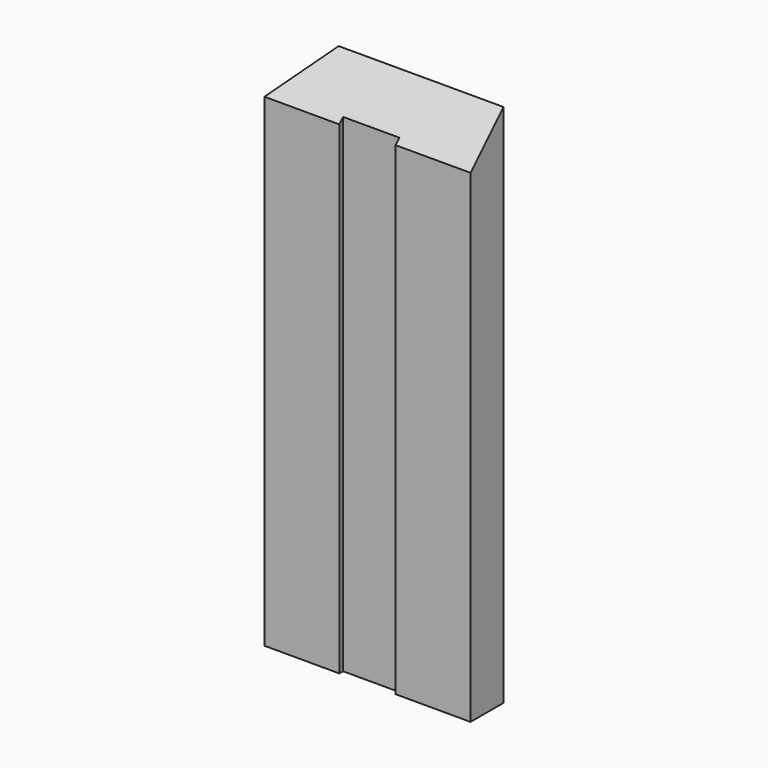
from build123d import *

# Parameters (mm, degrees)
F0_W     = 139.7
F0_H     = 27.94
F1_DEPTH = 355.6
F2_SIZE  = 27.93999
F3_W     = 38.1
F3_H     = 355.6
F4_DEPTH = 3.175
F6_DEPTH = 38.1


# Not quite as in the source:
# - a fillet or chamfer is up to 0.001 mm smaller than in the source, because OpenCascade refuses the exact size


with BuildPart() as f1:
    # F0 (on Top) → F1 (new body)
    with BuildSketch(Plane.XY):
        with Locations((69.85, -13.97)):
            Rectangle(F0_W, F0_H)
    extrude(amount=F1_DEPTH)

    # F2 (size 27.94 in the source; OpenCascade refuses exactly that, so slightly less here)
    f2_edges = [f1.edges().sort_by_distance(p)[0] for p in [
        (69.85, -27.94, 355.6),
    ]]
    chamfer(f2_edges, length=F2_SIZE)

    # F3 (on face) → F4 (cut)
    with BuildSketch(Plane.XZ.offset(27.94)):
        with Locations((69.85, 177.8)):
            Rectangle(F3_W, F3_H)
    extrude(amount=-F4_DEPTH, mode=Mode.SUBTRACT)

    # F5 (on face) → F6 (cut)
    with BuildSketch(Plane(origin=(0, 0, 0), x_dir=(-1, 0, 0), z_dir=(0, 1, 0))):
        Polygon((0, 327.66), (0, 355.6), (-27.94, 355.6), align=None)
    extrude(amount=-F6_DEPTH, mode=Mode.SUBTRACT)


solid = f1.part
